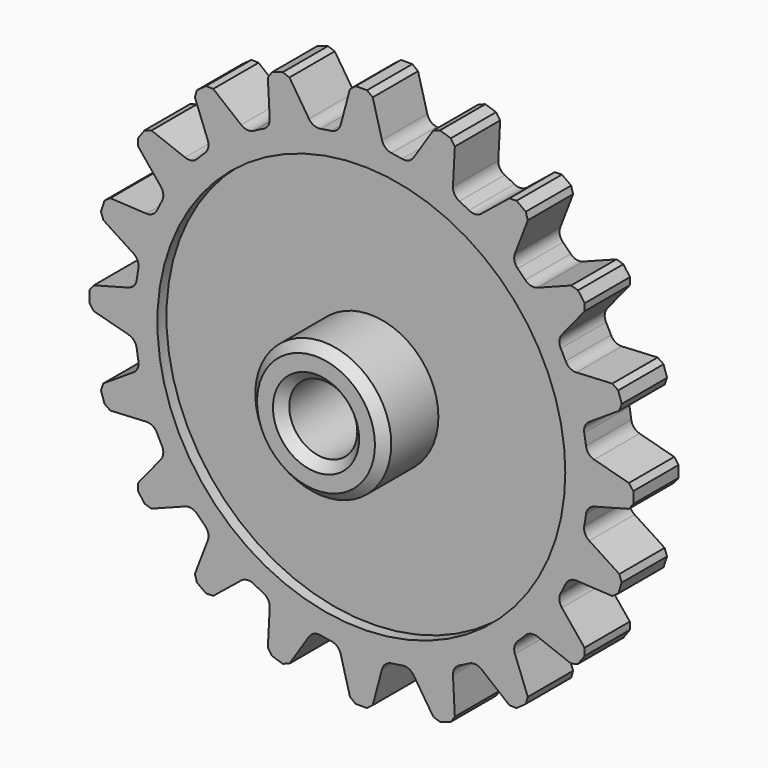
from build123d import *

# Parameters (mm, degrees)
F0_R            = 100
F1_DEPTH        = 25
F3_DEPTH        = 25
F3_COPIES_COUNT = 20
F4_R            = 5
F5_SIZE         = 2
F6_R            = 90
F7_DEPTH        = 5
F8_R            = 30
F9_DEPTH        = 30
F10_R           = 15
F11_DEPTH       = 50.001
F12_SIZE        = 4


# Not quite as in the source:
# - a pattern or mirror of a feature is missing from the dataset's text; its kind, count and spacing are read off the source's solid
# - a feature names something its author has since deleted; it is built from what else it names


with BuildPart() as f1:
    # F0 (on Front) → F1 (new body)
    with BuildSketch(Plane.XZ):
        Circle(F0_R)
    extrude(amount=F1_DEPTH)

    # F2 (on face) → F3 (join, through all)
    with BuildSketch(Plane.XZ.offset(25)):
        with BuildLine():
            Line((-4.5, 120), (-9.9931095726, 99.4994359837))
            ThreePointArc((-9.9931095726, 99.4994359837), (0, 100), (9.9931095726, 99.4994359837))
            Line((9.9931095726, 99.4994359837), (4.5, 120))
            Line((4.5, 120), (-4.5, 120))
        make_face()
    f3 = extrude(amount=-F3_DEPTH)

    # F3_copies: F3 ×20 about axis
    f3_copies_axis = Axis((0, 0, 0), (0, 1, 0))
    for i in range(1, F3_COPIES_COUNT):
        add(f3.rotate(f3_copies_axis, i * 360 / F3_COPIES_COUNT))

    # F4
    f4_edges = [f1.edges().sort_by_distance(p)[0] for p in [
        (9.99311, -12.5, 99.499436),
        (-9.99311, -12.5, 99.499436),
        (-21.243005, -12.5, 97.717628),
        (-50.399706, -12.5, 86.370537),
        (-40.251029, -12.5, 91.541546),
        (-66.568897, -12.5, 74.622932),
        (-74.622932, -12.5, 66.568897),
        (-86.370537, -12.5, 50.399706),
        (-91.541546, -12.5, 40.251029),
        (-97.717628, -12.5, 21.243005),
        (-99.499436, -12.5, 9.99311),
        (-99.499436, -12.5, -9.99311),
        (-97.717628, -12.5, -21.243005),
        (-91.541546, -12.5, -40.251029),
        (-86.370537, -12.5, -50.399706),
        (-74.622932, -12.5, -66.568897),
        (-66.568897, -12.5, -74.622932),
        (-50.399706, -12.5, -86.370537),
        (-40.251029, -12.5, -91.541546),
        (-21.243005, -12.5, -97.717628),
        (-9.99311, -12.5, -99.499436),
        (9.99311, -12.5, -99.499436),
        (21.243005, -12.5, -97.717628),
        (40.251029, -12.5, -91.541546),
        (50.399706, -12.5, -86.370537),
        (66.568897, -12.5, -74.622932),
        (74.622932, -12.5, -66.568897),
        (86.370537, -12.5, -50.399706),
        (91.541546, -12.5, -40.251029),
        (97.717628, -12.5, -21.243005),
        (99.499436, -12.5, -9.99311),
        (99.499436, -12.5, 9.99311),
        (97.717628, -12.5, 21.243005),
        (91.541546, -12.5, 40.251029),
        (86.370537, -12.5, 50.399706),
        (74.622932, -12.5, 66.568897),
        (66.568897, -12.5, 74.622932),
        (50.399706, -12.5, 86.370537),
        (40.251029, -12.5, 91.541546),
        (21.243005, -12.5, 97.717628),
    ]]
    fillet(f4_edges, radius=F4_R)

    # F5
    f5_edges = [f1.edges().sort_by_distance(p)[0] for p in [
        (4.5, -12.5, 120),
        (-4.5, -12.5, 120),
        (32.802285, -12.5, 115.517358),
        (41.361794, -12.5, 112.736205),
        (-32.802285, -12.5, 115.517358),
        (-41.361794, -12.5, 112.736205),
        (66.893654, -12.5, 99.727073),
        (74.174807, -12.5, 94.437006),
        (-66.893654, -12.5, 99.727073),
        (-74.174807, -12.5, 94.437006),
        (94.437006, -12.5, 74.174807),
        (99.727073, -12.5, 66.893654),
        (-94.437006, -12.5, 74.174807),
        (-99.727073, -12.5, 66.893654),
        (112.736205, -12.5, 41.361794),
        (115.517358, -12.5, 32.802285),
        (-112.736205, -12.5, 41.361794),
        (-115.517358, -12.5, 32.802285),
        (120, -12.5, 4.5),
        (120, -12.5, -4.5),
        (-120, -12.5, 4.5),
        (-120, -12.5, -4.5),
        (115.517358, -12.5, -32.802285),
        (112.736205, -12.5, -41.361794),
        (-115.517358, -12.5, -32.802285),
        (-112.736205, -12.5, -41.361794),
        (99.727073, -12.5, -66.893654),
        (94.437006, -12.5, -74.174807),
        (-99.727073, -12.5, -66.893654),
        (-94.437006, -12.5, -74.174807),
        (74.174807, -12.5, -94.437006),
        (66.893654, -12.5, -99.727073),
        (-74.174807, -12.5, -94.437006),
        (-66.893654, -12.5, -99.727073),
        (41.361794, -12.5, -112.736205),
        (32.802285, -12.5, -115.517358),
        (-41.361794, -12.5, -112.736205),
        (-32.802285, -12.5, -115.517358),
        (4.5, -12.5, -120),
        (-4.5, -12.5, -120),
    ]]
    chamfer(f5_edges, length=F5_SIZE)

    # F6 (on face) → F7 (cut)
    with BuildSketch(Plane.XZ.offset(25)):
        Circle(F6_R)
    extrude(amount=-F7_DEPTH, mode=Mode.SUBTRACT)

    # F8 (on face) → F9 (join)
    with BuildSketch(Plane.XZ.offset(20)):
        Circle(F8_R)
    extrude(amount=F9_DEPTH)

    # F10 (on face) → F11 (cut, through all)
    with BuildSketch(Plane.XZ.offset(50)):
        Circle(F10_R)
    extrude(amount=-F11_DEPTH, mode=Mode.SUBTRACT)

    # F12
    f12_edges = [f1.edges().sort_by_distance(p)[0] for p in [
        (-30, -50, 0),
        (-15, -50, 0),
    ]]
    chamfer(f12_edges, length=F12_SIZE)


solid = f1.part
